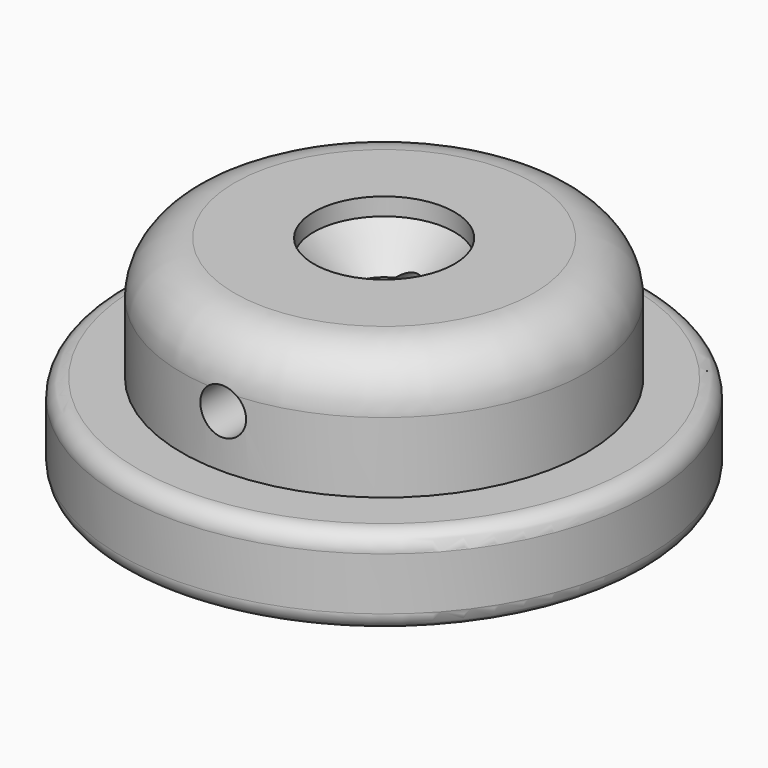
from build123d import *

# Parameters (mm, degrees)
F0_R           = 15
F0_R_2         = 11.5
F1_DEPTH       = 5
F0_R_3         = 2
F2_DEPTH       = 12
F3_R           = 3
F4_R           = 1
F5_R           = 4
F6_DEPTH       = 1
F7_SIZE        = 1.99999
F8_R           = 1.3
F9_DEPTH       = 25
F9_DEPTH_BACK  = 25
F10_W          = 6
F10_H          = 6
F11_DEPTH      = 5
F11_DEPTH_BACK = 2
F12_R          = 2
F13_DEPTH      = 25
F13_DEPTH_BACK = 25


# Not quite as in the source:
# - a fillet or chamfer is up to 0.001 mm smaller than in the source, because OpenCascade refuses the exact size


with BuildPart() as f1:
    # F0 (on Top) → F1 (new body)
    with BuildSketch(Plane.XY):
        Circle(F0_R)
        Circle(F0_R_2, mode=Mode.SUBTRACT)
    extrude(amount=F1_DEPTH)

    # F0 (on Top) → F2 (join)
    with BuildSketch(Plane.XY):
        Circle(F0_R_2)
        Circle(F0_R_3, mode=Mode.SUBTRACT)
    extrude(amount=F2_DEPTH)

    # F3
    f3_edges = [f1.edges().sort_by_distance(p)[0] for p in [
        (-11.5, 0, 12),
    ]]
    fillet(f3_edges, radius=F3_R)

    # F4
    f4_edges = [f1.edges().sort_by_distance(p)[0] for p in [
        (-15, 0, 0),
        (-15, 0, 5),
    ]]
    fillet(f4_edges, radius=F4_R)

    # F5 (on face) → F6 (cut)
    with BuildSketch(Plane.XY.offset(12)):
        Circle(F5_R)
    extrude(amount=-F6_DEPTH, mode=Mode.SUBTRACT)

    # F7 (size 2 in the source; OpenCascade refuses exactly that, so slightly less here)
    f7_edges = [f1.edges().sort_by_distance(p)[0] for p in [
        (-2, 0, 11),
    ]]
    chamfer(f7_edges, length=F7_SIZE)

    # F8 (on Front) → F9 (cut, two sides)
    with BuildSketch(Plane.XZ) as f9_sk:
        with Locations((0, 8)):
            Circle(F8_R)
    extrude(amount=F9_DEPTH, mode=Mode.SUBTRACT)
    extrude(f9_sk.sketch, amount=-F9_DEPTH_BACK, mode=Mode.SUBTRACT)

    # F10 (on Top) → F11 (join, two sides)
    with BuildSketch(Plane.XY) as f11_sk:
        Rectangle(F10_W, F10_H)
    extrude(amount=F11_DEPTH)
    extrude(f11_sk.sketch, amount=-F11_DEPTH_BACK)

    # F12 (on Top) → F13 (cut, two sides)
    with BuildSketch(Plane.XY) as f13_sk:
        Circle(F12_R)
    extrude(amount=-F13_DEPTH, mode=Mode.SUBTRACT)
    extrude(f13_sk.sketch, amount=F13_DEPTH_BACK, mode=Mode.SUBTRACT)


solid = f1.part
